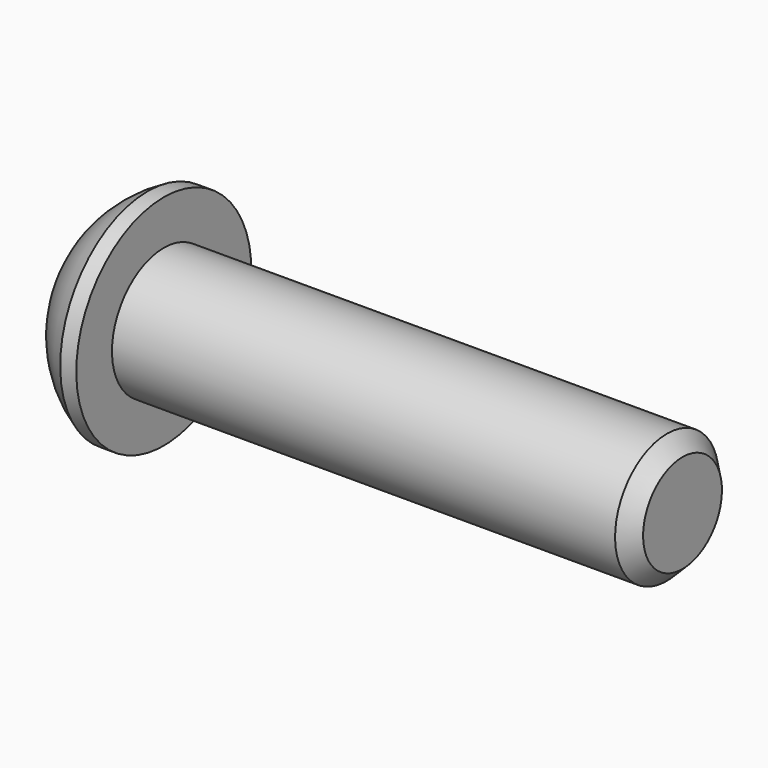
from build123d import *

# Parameters (mm, degrees)
F0_W     = 25.4
F0_H     = 3.175
F3_DEPTH = 2.8194
F4_SIZE2 = 0.762
F4_SIZE  = 0.762


# Not quite as in the source:
# - a feature names something its author has since deleted; it is built from what else it names


with BuildPart() as f1:
    # F0 (on Front) → F1 (revolve)
    with BuildSketch(Plane.XZ):
        with Locations((12.7, 1.5875)):
            Rectangle(F0_W, F0_H)
        with BuildLine():
            Line((-3.175, 0), (0, 0))
            Line((0, 0), (0, 3.175))
            Line((0, 3.175), (0, 5.3594))
            Line((0, 5.3594), (-0.7874, 5.3594))
            ThreePointArc((-0.7874, 5.3594), (-2.1313938593, 4.4313653811), (-3.175, 3.175))
            Line((-3.175, 3.175), (-3.175, 0))
        make_face()
    revolve(axis=Axis((12.7, 0, 0), (1, 0, 0)))

    # F2 (on face) → F3 (cut)
    with BuildSketch(Plane(origin=(-3.175, 0, 0), x_dir=(0, -1, 0), z_dir=(-1, 0, 0))):
        Polygon((1.9122612153, 1.2623718016), (-0.1371154416, 2.2872526919), (-2.0493766568, 1.0248808903), (-1.9122612153, -1.2623718016), (0.1371154416, -2.2872526919), (2.0493766568, -1.0248808903), align=None)
    extrude(amount=-F3_DEPTH, mode=Mode.SUBTRACT)

    # F4
    f4_edges = [f1.edges().sort_by_distance(p)[0] for p in [
        (25.4, 0, -3.175),
    ]]
    chamfer(f4_edges, length=F4_SIZE, length2=F4_SIZE2)


solid = f1.part
